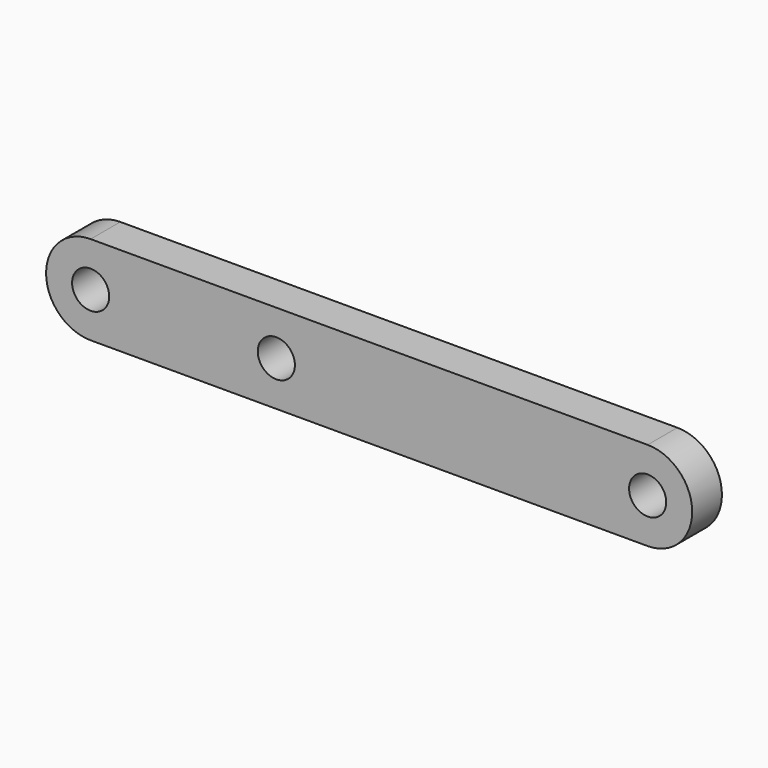
from build123d import *

# Parameters (mm, degrees)
F0_R     = 2.5
F1_DEPTH = 5


# Not quite as in the source:
# - a feature names something its author has since deleted; it is built from what else it names


with BuildPart() as f1:
    # F0 (on Front) → F1 (new body)
    with BuildSketch(Plane.XZ):
        with BuildLine():
            ThreePointArc((0, 12), (-6, 6), (0, 0))
            Line((0, 0), (75, 0))
            ThreePointArc((75, 0), (81, 6), (75, 12))
            Line((75, 12), (0, 12))
        make_face()
        with Locations((0, 6)):
            Circle(F0_R, mode=Mode.SUBTRACT)
        with Locations((25, 6)):
            Circle(F0_R, mode=Mode.SUBTRACT)
        with Locations((75, 6)):
            Circle(F0_R, mode=Mode.SUBTRACT)
    extrude(amount=F1_DEPTH)


solid = f1.part
